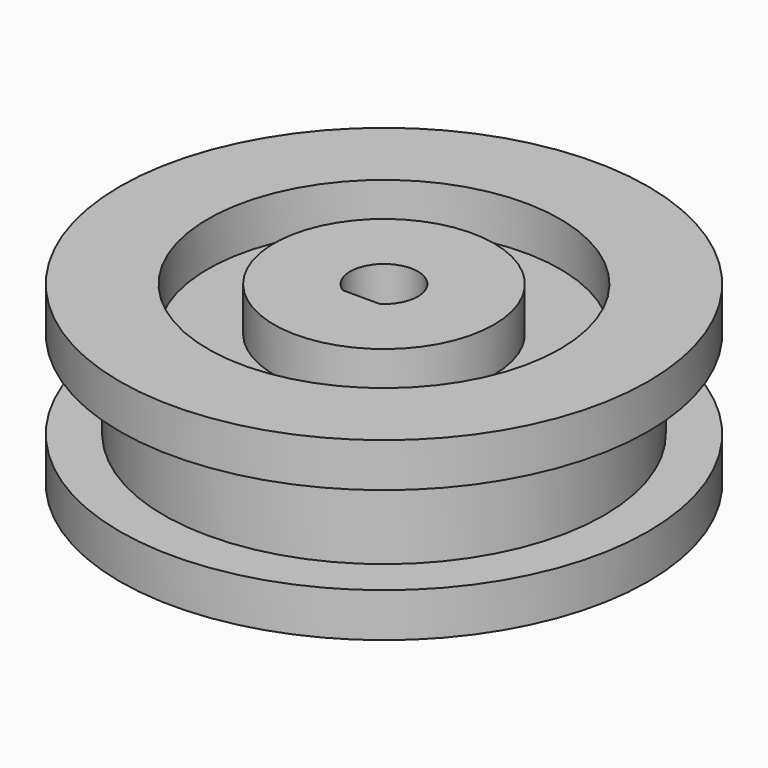
from build123d import *

# Parameters (mm, degrees)
F0_R      = 19.05
F1_DEPTH  = 3.175
F2_R      = 15.875
F3_DEPTH  = 6.35
F4_R      = 19.05
F5_DEPTH  = 3.175
F6_R      = 12.7
F6_R_2    = 7.9375
F7_DEPTH  = 3.175
F10_DEPTH = 12.7


# Not quite as in the source:
# - a pattern or mirror of a feature is missing from the dataset's text; its kind, count and spacing are read off the source's solid


with BuildPart() as f1:
    # F0 (on Top) → F1 (new body)
    with BuildSketch(Plane.XY):
        Circle(F0_R)
    extrude(amount=F1_DEPTH)

    # F2 (on face) → F3 (join)
    with BuildSketch(Plane.XY.offset(3.175)):
        Circle(F2_R)
    extrude(amount=F3_DEPTH)

    # F4 (on face) → F5 (join)
    with BuildSketch(Plane.XY.offset(9.525)):
        Circle(F4_R)
    extrude(amount=F5_DEPTH)

    # F6 (on face) → F7 (cut)
    with BuildSketch(Plane.XY.offset(12.7)):
        Circle(F6_R)
        Circle(F6_R_2, mode=Mode.SUBTRACT)
    f7 = extrude(amount=-F7_DEPTH, mode=Mode.SUBTRACT)

    # F7_copies: F7 across plane
    add(f7.mirror(Plane(origin=(0, 0, 6.35), x_dir=(-1, 0, 0), z_dir=(0, 0, -1))), mode=Mode.SUBTRACT)

    # F9 (on face) → F10 (cut, through all)
    with BuildSketch(Plane.XY.offset(12.7)):
        with BuildLine():
            Line((-1.3352941799, -2.047875), (1.3352941799, -2.047875))
            ThreePointArc((1.3352941799, -2.047875), (0, 2.44475), (-1.3352941799, -2.047875))
        make_face()
    extrude(amount=-F10_DEPTH, mode=Mode.SUBTRACT)


solid = f1.part
